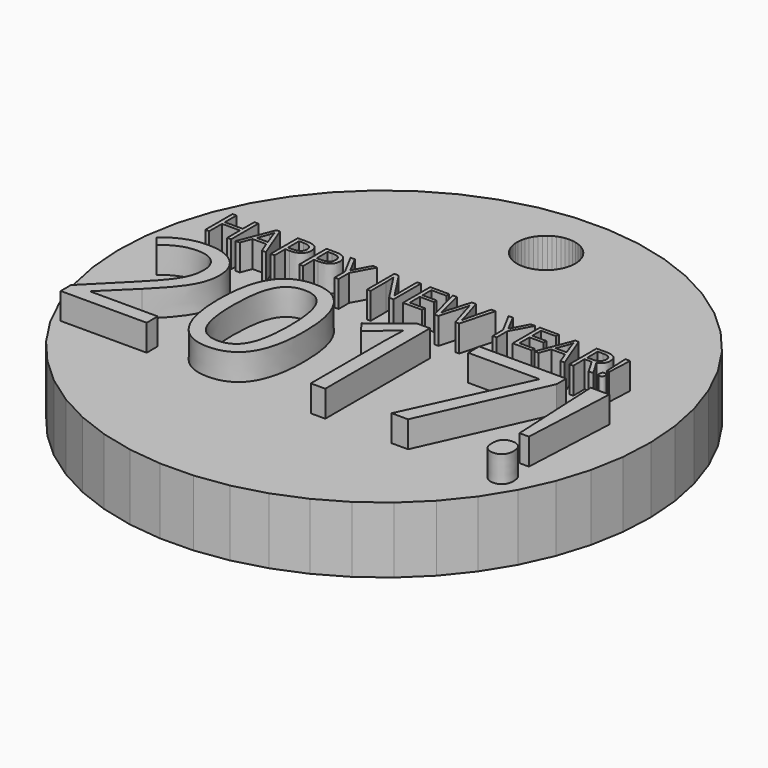
from build123d import *

# Parameters (mm, degrees)
F1_DEPTH       = 6.35
F2_TEXT_SIZE   = 17.6329792097
F2_TEXT_SIZE_2 = 4.5852664559
F3_DEPTH       = 2.54
F5_DEPTH       = 25.4


# Not quite as in the source:
# - Text() gives the source's letters only with a copy of the font that has no kerning and outlines rounded to 1/6400 em; it was checked with that copy


with BuildPart() as f1:
    # F0 (on Top) → F1 (new body)
    with BuildSketch(Plane.XY):
        Polygon((23.4845250305, 9.6766256563), (22.0865397526, 12.5437140336), (20.340236549, 15.2129805472), (18.2731556643, 17.6423292699), (15.917896199, 19.7934479209), (13.3116020017, 21.6324120742), (10.4953758889, 23.1302201665), (7.5136314287, 24.2632508695), (4.4133925124, 25.013635612), (1.2435517598, 25.3695403786), (-1.945900547, 25.3253523383), (-5.1046648397, 24.8817683631), (-8.1829255185, 24.0457840371), (-11.1321365736, 22.8305833326), (-13.9057871849, 21.2553306906), (-16.4601352255, 19.3448687863), (-18.7548971007, 17.1293267452), (-20.753883045, 14.6436449887), (-22.4255678559, 11.9270242031), (-23.7435880653, 9.0223071209), (-24.6871577072, 5.9753028658), (-25.2413961247, 2.834064515), (-25.3975626468, -0.3518687262), (-25.1531944342, -3.5322527873), (-24.5121453196, -6.656931112), (-23.4845250305, -9.6766256563), (-22.0865397526, -12.5437140336), (-20.340236549, -15.2129805472), (-18.2731556643, -17.6423292699), (-15.917896199, -19.7934479209), (-13.3116020017, -21.6324120742), (-10.4953758889, -23.1302201665), (-7.5136314287, -24.2632508695), (-4.4133925124, -25.013635612), (-1.2435517598, -25.3695403786), (1.945900547, -25.3253523383), (5.1046648397, -24.8817683631), (8.1829255185, -24.0457840371), (11.1321365736, -22.8305833326), (13.9057871849, -21.2553306906), (16.4601352255, -19.3448687863), (18.7548971007, -17.1293267452), (20.753883045, -14.6436449887), (22.4255678559, -11.9270242031), (23.7435880653, -9.0223071209), (24.6871577072, -5.9753028658), (25.2413961247, -2.834064515), (25.3975626468, 0.3518687262), (25.1531944342, 3.5322527873), (24.5121453196, 6.656931112), align=None)
    extrude(amount=F1_DEPTH)

    # F2 (on face) → F3 (join)
    with BuildSketch(Plane.XY.offset(6.35)):
        with Locations((-22.4255678559, -11.9270242031)):
            Text('2017!', F2_TEXT_SIZE, font='Open Sans', text_align=(TextAlign.LEFT, TextAlign.BOTTOM))
        with Locations((-19.7543900728, 2.6355246399)):
            Text('HAPPY NEW YEAR!', F2_TEXT_SIZE_2, font='Open Sans', text_align=(TextAlign.LEFT, TextAlign.BOTTOM))
    extrude(amount=F3_DEPTH)

    # F4 (on face) → F5 (cut)
    with BuildSketch(Plane.XY.offset(6.35)):
        Polygon((2.5141485733, 20.7227051919), (2.3406075779, 21.0281405598), (2.1301538029, 21.3094170244), (1.8861062299, 21.562098688), (1.612313635, 21.7822006097), (1.3130938908, 21.9662516508), (0.9931658717, 22.1113492163), (0.6575750334, 22.2152050311), (0.311613844, 22.2761812268), (-0.0392616818, 22.2933161725), (-0.3895180275, 22.2663396398), (-0.7336314411, 22.1956770647), (-1.0661750487, 22.0824428382), (-1.3819044389, 21.9284227319), (-1.6758403706, 21.7360457346), (-1.9433472985, 21.5083457467), (-2.1802064786, 21.2489137329), (-2.3826825002, 20.9618410911), (-2.5475821954, 20.6516551283), (-2.6723049975, 20.3232476625), (-2.7548839534, 19.9817978755), (-2.7940167438, 19.6326906345), (-2.789086221, 19.2814315692), (-2.7401701424, 18.933560245), (-2.6480399437, 18.5945628003), (-2.5141485733, 18.2697854275), (-2.3406075779, 17.9643500596), (-2.1301538029, 17.683073595), (-1.8861062299, 17.4303919314), (-1.612313635, 17.2102900097), (-1.3130938908, 17.0262389686), (-0.9931658717, 16.8811414031), (-0.6575750334, 16.7772855883), (-0.311613844, 16.7163093926), (0.0392616818, 16.6991744469), (0.3895180275, 16.7261509797), (0.7336314411, 16.7968135547), (1.0661750487, 16.9100477812), (1.3819044389, 17.0640678876), (1.6758403706, 17.2564448848), (1.9433472985, 17.4841448727), (2.1802064786, 17.7435768865), (2.3826825002, 18.0306495283), (2.5475821954, 18.3408354911), (2.6723049975, 18.669242957), (2.7548839534, 19.0106927439), (2.7940167438, 19.3597999849), (2.789086221, 19.7110590502), (2.7401701424, 20.0589303744), (2.6480399437, 20.3979278191), align=None)
    extrude(amount=-F5_DEPTH, mode=Mode.SUBTRACT)


solid = f1.part
